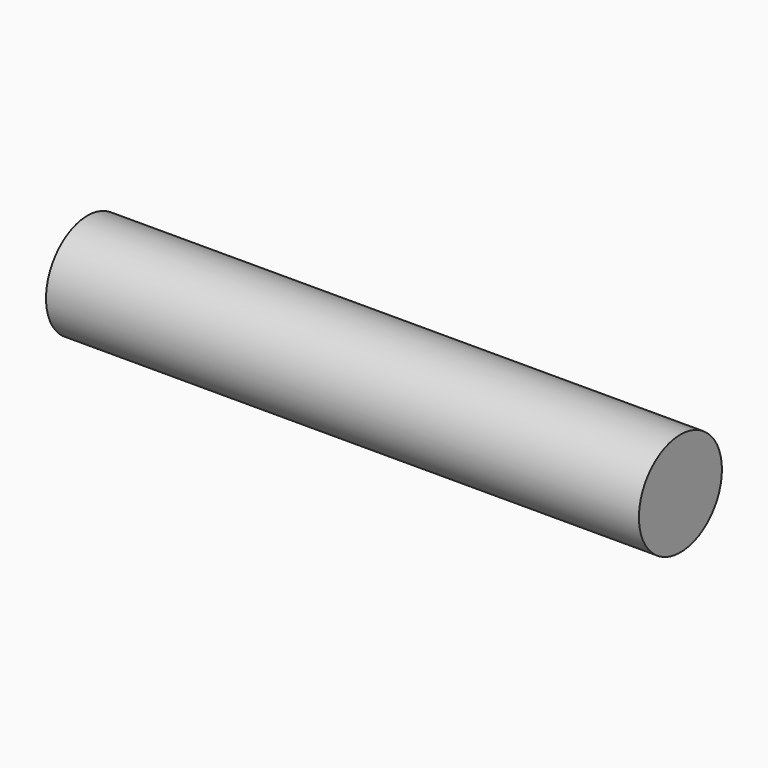
from build123d import *

# Parameters (mm, degrees)
F0_R     = 7
F1_DEPTH = 40


# Not quite as in the source:
# - the program builds the solid bodies; features that only make, move or delete a surface that nothing else refers to are left out


with BuildPart() as f1:
    # F0 (on Right) → F1 (new body, symmetric)
    with BuildSketch(Plane.YZ):
        Circle(F0_R)
    extrude(amount=F1_DEPTH, both=True)


solid = f1.part
